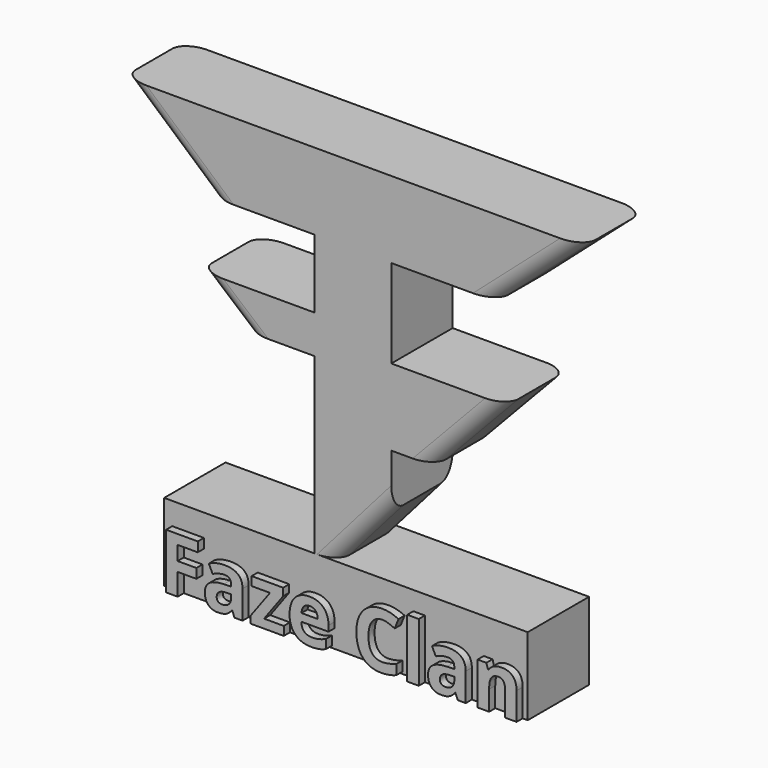
from build123d import *

# Parameters (mm, degrees)
F1_DEPTH     = 25.4
F2_R         = 5.08
F3_W         = 120.452132076
F3_H         = 25.6841517985
F4_DEPTH     = 25.4
F5_TEXT_SIZE = 25.6315256533
F6_DEPTH     = 2.54


# Not quite as in the source:
# - Text() gives the source's letters only with a copy of the font that has no kerning and outlines rounded to 1/6400 em; it was checked with that copy


with BuildPart() as f1:
    # F0 (on Front) → F1 (new body)
    with BuildSketch(Plane.XZ):
        Polygon((-47.6203486323, 42.2727518439), (-13.1124399222, 42.2727518439), (-13.1124399222, 19.5496726453), (-13.1124399222, 6.8496726453), (-13.1124399222, -59.3272481561), (12.2875600778, -30.3267855197), (12.2875600778, -12.4293438435), (12.2875600778, 12.9706561565), (12.2875600778, 42.2727518439), (47.0328070223, 42.2727518439), (75.9087558627, 67.6727518439), (-76.4912441373, 67.6727518439), align=None)
        Polygon((-13.1124399222, 6.8496726453), (-13.1124399222, 19.5496726453), (-51.2124399222, 19.5496726453), (-36.2762138247, 6.8496726453), align=None)
        Polygon((12.2875600778, 12.9706561565), (12.2875600778, -12.4293438435), (26.3786390424, -12.4293438435), (50.3875600778, 12.9706561565), align=None)
    extrude(amount=F1_DEPTH)

    # F2
    f2_edges = [f1.edges().sort_by_distance(p)[0] for p in [
        (-62.055796, -25.4, 54.972752),
        (61.470781, -25.4, 54.972752),
        (38.3831, -25.4, 0.270656),
        (-43.744327, -25.4, 13.199673),
        (-0.41244, -25.4, -44.827017),
        (-43.744327, 0, 13.199673),
        (-62.055796, 0, 54.972752),
        (61.470781, 0, 54.972752),
        (38.3831, 0, 0.270656),
        (-0.41244, 0, -44.827017),
    ]]
    fillet(f2_edges, radius=F2_R)

    # F3 (on face) → F4 (join)
    with BuildSketch(Plane.XZ.offset(25.4)):
        with Locations((-2.7406532317, -63.5367203504)):
            Rectangle(F3_W, F3_H)
    extrude(amount=-F4_DEPTH)

    # F5 (on face) → F6 (join)
    with BuildSketch(Plane.XZ.offset(25.4)):
        with Locations((-62.5902750277, -76.3787962496)):
            Text('Faze Clan', F5_TEXT_SIZE, font='Open Sans', font_style=FontStyle.BOLD, text_align=(TextAlign.LEFT, TextAlign.BOTTOM))
    extrude(amount=F6_DEPTH)


solid = f1.part
